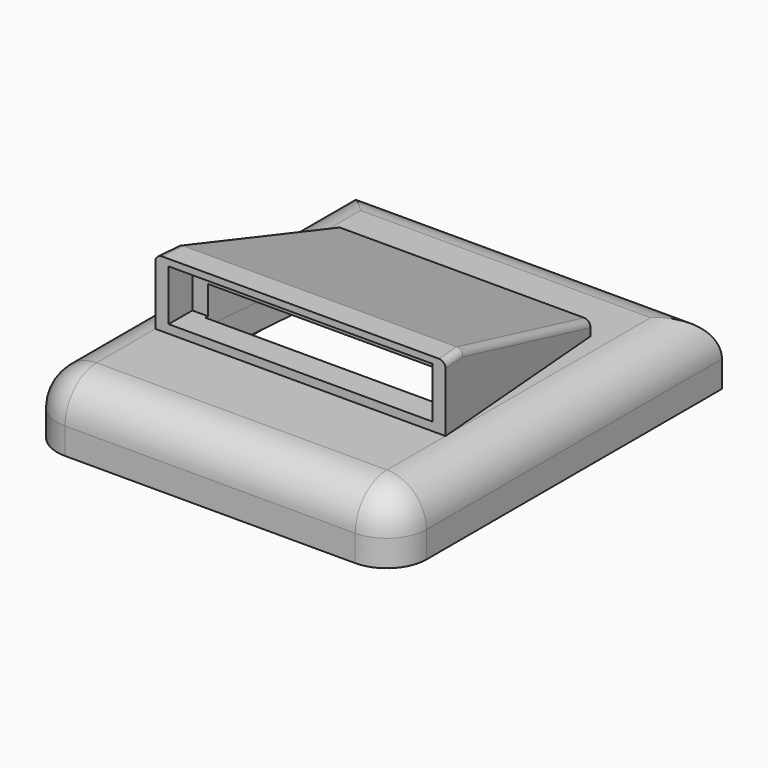
from build123d import *

# Parameters (mm, degrees)
F0_W         = 560
F0_H         = 620
F1_DEPTH     = 100
F2_R         = 60
F3_R         = 60
F5_DEPTH     = 100
F7_DEPTH     = 560.001
F8_R         = 10
F10_T        = 40
F10_T3_DEPTH = 520
F10_T5_DEPTH = 388.1889053137
F10_T7_DEPTH = 388.1889053137
F10_T9_DEPTH = 468.2577419281
F9_W         = 399.9291565789
F9_H         = 77.1599882841
F11_DEPTH    = 45


# Not quite as in the source:
# - a shell that OpenCascade refuses in one call is made with other operations: the cavity is built on its own and cut out


with BuildPart() as f1:
    # F0 (on Top) → F1 (new body)
    with BuildSketch(Plane.XY):
        Rectangle(F0_W, F0_H)
    extrude(amount=F1_DEPTH)

    # F2
    f2_edges = [f1.edges().sort_by_distance(p)[0] for p in [
        (280, -310, 50),
        (-280, -310, 50),
    ]]
    fillet(f2_edges, radius=F2_R)

    # F3
    f3_edges = [f1.edges().sort_by_distance(p)[0] for p in [
        (0, -310, 100),
        (-262.426407, -292.426407, 100),
        (262.426407, -292.426407, 100),
        (-280, 30, 100),
        (280, 30, 100),
        (0, 310, 100),
    ]]
    fillet(f3_edges, radius=F3_R)

    # F4 (on face) → F5 (join)
    with BuildSketch(Plane.XY.offset(100)):
        Polygon((-194.1288709641, 168.3533191681), (-220, -138.7477815151), (0, -138.7477815151), (220, -138.7477815151), (194.1288709641, 168.3533191681), (0, 168.3533191681), align=None)
    extrude(amount=F5_DEPTH)

    # F6 (on face) → F7 (cut, through all)
    with BuildSketch(Plane.YZ.offset(280)):
        Polygon((261.031751243, 237.4019711016), (-149.0081892093, 213.623028462), (222.8016257286, 105.6972444057), align=None)
    extrude(amount=-F7_DEPTH, mode=Mode.SUBTRACT)

    # F8
    f8_edges = [f1.edges().sort_by_distance(p)[0] for p in [
        (218.455336, -120.411972, 200),
        (205.519771, 33.138578, 160.751017),
        (-218.455336, -120.411972, 200),
        (-205.519771, 33.138578, 160.751017),
    ]]
    fillet(f8_edges, radius=F8_R)

    # F10: shell of thickness 40, made by hand


with BuildPart() as f10_core1:
    # F10_t2: copy of F1
    add(f1.part)

    # the walls: a layer under each face that stays
    f10_faces = [f10_core1.faces().sort_by_distance(p)[0] for p in [
        (0, -138.7477815151, 150),
        (-207.064435482, 14.8027688265, 145),
        (0, -194.3738907576, 100),
        (0, -120.411972418, 200),
        (207.064435482, 14.8027688265, 145),
        (-146.6666666667, 185.2087030808, 100),
        (0, 168.3533191681, 110.7510173791),
        (0, 33.1385779236, 160.7510173791),
        (262.4264068712, 30, 82.4264068712),
        (0, -292.4264068712, 82.4264068712),
        (-262.4264068712, 30, 82.4264068712),
        (0, 292.4264068712, 82.4264068712),
        (250, -280, 82.4264068712),
        (280, 30, 20),
        (-250, -280, 82.4264068712),
        (0, -310, 20),
        (-280, 30, 20),
        (0, 310, 20),
        (262.4264068712, -292.4264068712, 20),
        (-262.4264068712, -292.4264068712, 20),
    ]]
    thicken(f10_faces, amount=-F10_T, mode=Mode.SUBTRACT)

    # F10_s4 → F10_t3 (cut)
    with BuildSketch(Plane.YZ.offset(-260)):
        Polygon((-139.1477815151, 100.4), (-98.7477815151, 100), (-98.7477815151, 60), (-138.7477815151, 60), align=None)
    extrude(amount=F10_T3_DEPTH, mode=Mode.SUBTRACT)

    # F10_s6 → F10_t5 (cut)
    with BuildSketch(Plane(origin=(16.0724766165, 190.7870063494, 0), x_dir=(0, 0, 1), z_dir=(-0.0839456859, -0.9964703316, 0))):
        Polygon((100.4, 207.976195276), (100, 167.576195276), (60, 167.576195276), (60, 207.576195276), align=None)
    extrude(amount=F10_T5_DEPTH, mode=Mode.SUBTRACT)

    # F10_s8 → F10_t7 (cut)
    with BuildSketch(Plane(origin=(16.5143072895, -196.0317208644, 0), x_dir=(0, 0, 1), z_dir=(-0.0839456859, 0.9964703316, 0))):
        Polygon((100.4, 207.976195276), (100, 167.576195276), (60, 167.576195276), (60, 207.576195276), align=None)
    extrude(amount=F10_T7_DEPTH, mode=Mode.SUBTRACT)

    # F10_s10 → F10_t9 (cut)
    with BuildSketch(Plane.YZ.offset(-234.1288709641)):
        Polygon((168.7533191681, 100.4), (168.3533191681, 60), (128.3533191681, 60), (128.3533191681, 100), align=None)
    extrude(amount=F10_T9_DEPTH, mode=Mode.SUBTRACT)


with BuildPart() as f1_1:
    add(f1.part)

    # what is left inside the walls is the cavity
    f10_cavity = [f10_core1.part.solids().sort_by_distance(p)[0] for p in [
        (0, -90, 0.4),
    ]]
    add(f10_cavity, mode=Mode.SUBTRACT)

    # F9 (on face) → F11 (cut)
    with BuildSketch(Plane.XZ.offset(138.7477815151)):
        with Locations((0.0354217106, 151.4200058579)):
            Rectangle(F9_W, F9_H)
    extrude(amount=-F11_DEPTH, mode=Mode.SUBTRACT)


solid = f1_1.part
